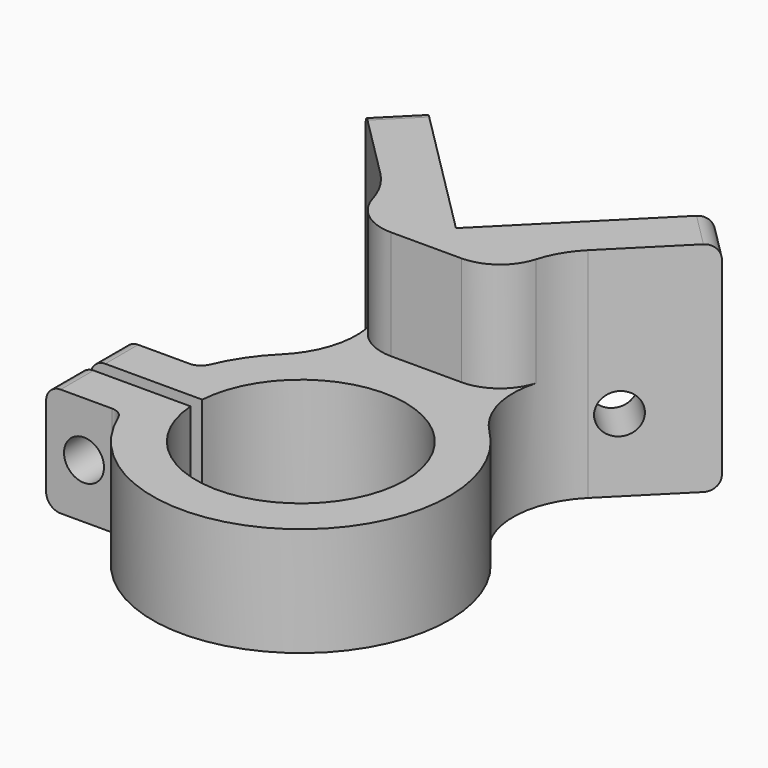
from build123d import *

# Parameters (mm, degrees)
F1_DEPTH      = 45
F2_R          = 4.125
F3_DEPTH      = 10
F4_R          = 4.125
F5_DEPTH      = 10
F6_R          = 4.125
F7_DEPTH      = 20
F9_DEPTH      = 3
F10_R         = 18
F11_W         = 72.4435358676
F11_H         = 36.0539390085
F12_DEPTH     = 100
F13_T1_DEPTH  = 22.5
F13_T6_DEPTH  = 22.5
F13_T12_DEPTH = 22.5
F13_T18_DEPTH = 22.5
F13_T25_DEPTH = 22.5
F13_T31_DEPTH = 22.5
F13_T34_DEPTH = 23.5
F13_T36_DEPTH = 23.5
F13_T38_DEPTH = 25
F13_T40_DEPTH = 25
F14_R         = 10


# Not quite as in the source:
# - a fillet or chamfer that OpenCascade refuses, or shapes differently, is made with other operations: its cross-section is extruded or revolved along the edge and cut away or added


with BuildPart() as f1:
    # F0 (on Top) → F1 (new body)
    with BuildSketch(Plane.XY):
        with BuildLine():
            Line((29.6984848098, 29.6984848098), (0, 0))
            Line((0, 0), (-29.6984848098, 29.6984848098))
            Line((-29.6984848098, 29.6984848098), (-36.7695526217, 22.627416998))
            Line((-36.7695526217, 22.627416998), (-4.4122546938, -9.7298809299))
            ThreePointArc((-4.4122546938, -9.7298809299), (-19.5013094439, -16.4320762481), (-28.9093081896, -30))
            ThreePointArc((-28.9093081896, -30), (-30.0334813831, -34.1915496034), (-30.5532011416, -38.5))
            Line((-30.5532011416, -38.5), (-21.53782951, -38.5))
            ThreePointArc((-21.53782951, -38.5), (21.59, -40), (-21.53782951, -41.5))
            Line((-21.53782951, -41.5), (-30.5532011416, -41.5))
            ThreePointArc((-30.5532011416, -41.5), (-30.0334813831, -45.8084503966), (-28.9093081896, -50))
            ThreePointArc((-28.9093081896, -50), (23.5679237519, -59.5013094439), (4.4122546938, -9.7298809299))
            Line((4.4122546938, -9.7298809299), (36.7695526217, 22.627416998))
            Line((36.7695526217, 22.627416998), (29.6984848098, 29.6984848098))
        make_face()
        with BuildLine():
            ThreePointArc((-30.5532011416, -38.5), (-30.0334813831, -34.1915496034), (-28.9093081896, -30))
            Line((-28.9093081896, -30), (-44.5532011416, -30))
            Line((-44.5532011416, -30), (-44.5532011416, -38.5))
            Line((-44.5532011416, -38.5), (-30.5532011416, -38.5))
        make_face()
        with BuildLine():
            Line((-44.5532011416, -50), (-28.9093081896, -50))
            ThreePointArc((-28.9093081896, -50), (-30.0334813831, -45.8084503966), (-30.5532011416, -41.5))
            Line((-30.5532011416, -41.5), (-44.5532011416, -41.5))
            Line((-44.5532011416, -41.5), (-44.5532011416, -50))
        make_face()
    extrude(amount=F1_DEPTH)

    # F2 (on face) → F3 (cut, through all)
    with BuildSketch(Plane(origin=(0, 0, 0), x_dir=(-0.7071067812, -0.7071067812, 0), z_dir=(-0.7071067812, 0.7071067812, 0))):
        with Locations((-25.4, 15)):
            Circle(F2_R)
    extrude(amount=-F3_DEPTH, mode=Mode.SUBTRACT)

    # F4 (on face) → F5 (cut, through all)
    with BuildSketch(Plane(origin=(0, 0, 0), x_dir=(-0.7071067812, 0.7071067812, 0), z_dir=(0.7071067812, 0.7071067812, 0))):
        with Locations((25.4, 15)):
            Circle(F4_R)
    extrude(amount=-F5_DEPTH, mode=Mode.SUBTRACT)

    # F6 (on face) → F7 (cut, through all)
    with BuildSketch(Plane.XZ.offset(50)):
        with Locations((-36.7312546656, 33.75)):
            Circle(F6_R)
        with Locations((-36.7312546656, 11.25)):
            Circle(F6_R)
    extrude(amount=-F7_DEPTH, mode=Mode.SUBTRACT)

    # F8 (on face) → F9 (cut)
    with BuildSketch(Plane(origin=(0, -30, 0), x_dir=(-1, 0, 0), z_dir=(0, 1, 0))):
        Polygon((43.6562546656, 37.7481506141), (36.7312546656, 41.7463012283), (29.8062546656, 37.7481506141), (29.8062546656, 29.7518493859), (36.7312546656, 25.7536987717), (43.6562546656, 29.7518493859), align=None)
        Polygon((43.6562546656, 7.2518493859), (43.6562546656, 15.2481506141), (36.7312546656, 19.2463012283), (29.8062546656, 15.2481506141), (29.8062546656, 7.2518493859), (36.7312546656, 3.2536987717), align=None)
    extrude(amount=-F9_DEPTH, mode=Mode.SUBTRACT)

    # F10
    f10_edges = [f1.edges().sort_by_distance(p)[0] for p in [
        (-4.412255, -9.729881, 22.5),
        (4.412255, -9.729881, 22.5),
    ]]
    fillet(f10_edges, radius=F10_R)

    # F11 (on Right) → F12 (cut, symmetric)
    with BuildSketch(Plane.YZ):
        with Locations((-43.9025410381, 40.5269695042)):
            Rectangle(F11_W, F11_H)
    extrude(amount=F12_DEPTH, both=True, mode=Mode.SUBTRACT)

    # F13: fillet of radius 3 on 10 edges, made by hand

    # F13_s2 → F13_t1 (join)
    with BuildSketch(Plane.XY):
        with BuildLine():
            ThreePointArc((-28.206162374, -51.8389401608), (-29.3115301597, -50.5016826145), (-30.9723764022, -50))
            Line((-30.9723764022, -50), (-28.9093081896, -50))
            ThreePointArc((-28.9093081896, -50), (-28.5725334833, -50.9251283904), (-28.206162374, -51.8389401608))
        make_face()
    extrude(amount=F13_T1_DEPTH)


with BuildPart() as f13_tool4:
    # F13_s5 → F13_t6 (new body)
    with BuildSketch(Plane.XY):
        with BuildLine():
            ThreePointArc((-28.206162374, -28.1610598392), (-29.3115301597, -29.4983173855), (-30.9723764022, -30))
            Line((-30.9723764022, -30), (-28.9093081896, -30))
            ThreePointArc((-28.9093081896, -30), (-28.5725334833, -29.0748716096), (-28.206162374, -28.1610598392))
        make_face()
    extrude(amount=F13_T6_DEPTH)

    split(bisect_by=Plane(origin=(-10.5917065627, 0, 18.3453739054), x_dir=(0, 1, 0), z_dir=(0.5, 0, -0.8660254038)), keep=Keep.TOP)

    split(bisect_by=Plane.YZ.offset(-29.8062546656), keep=Keep.TOP)


with BuildPart() as f1_1:
    add(f1.part)

    # F13_t3: union F13_tool4
    add(f13_tool4.part)


with BuildPart() as f13_tool10:
    # F13_s11 → F13_t12 (new body)
    with BuildSketch(Plane.XY):
        with BuildLine():
            ThreePointArc((-28.206162374, -28.1610598392), (-29.3115301597, -29.4983173855), (-30.9723764022, -30))
            Line((-30.9723764022, -30), (-28.9093081896, -30))
            ThreePointArc((-28.9093081896, -30), (-28.5725334833, -29.0748716096), (-28.206162374, -28.1610598392))
        make_face()
    extrude(amount=F13_T12_DEPTH)

    split(bisect_by=Plane(origin=(-10.5917065627, 0, 18.3453739054), x_dir=(0, 1, 0), z_dir=(0.5, 0, -0.8660254038)), keep=Keep.TOP)

    split(bisect_by=Plane.YZ.offset(-29.8062546656), keep=Keep.BOTTOM)


with BuildPart() as f1_2:
    add(f1_1.part)

    # F13_t9: union F13_tool10
    add(f13_tool10.part)


with BuildPart() as f13_tool16:
    # F13_s17 → F13_t18 (new body)
    with BuildSketch(Plane.XY):
        with BuildLine():
            ThreePointArc((-28.206162374, -28.1610598392), (-29.3115301597, -29.4983173855), (-30.9723764022, -30))
            Line((-30.9723764022, -30), (-28.9093081896, -30))
            ThreePointArc((-28.9093081896, -30), (-28.5725334833, -29.0748716096), (-28.206162374, -28.1610598392))
        make_face()
    extrude(amount=F13_T18_DEPTH)

    split(bisect_by=Plane(origin=(-10.5917065627, 0, 18.3453739054), x_dir=(0, 1, 0), z_dir=(-0.5, 0, 0.8660254038)), keep=Keep.TOP)

    split(bisect_by=Plane.YZ.offset(-29.8062546656), keep=Keep.TOP)

    split(bisect_by=Plane(origin=(-0.8489207701, 0, -1.4703739054), x_dir=(0, 1, 0), z_dir=(-0.5, 0, -0.8660254038)), keep=Keep.TOP)


with BuildPart() as f1_3:
    add(f1_2.part)

    # F13_t15: union F13_tool16
    add(f13_tool16.part)


with BuildPart() as f13_tool23:
    # F13_s24 → F13_t25 (new body)
    with BuildSketch(Plane.XY):
        with BuildLine():
            ThreePointArc((-28.206162374, -28.1610598392), (-29.3115301597, -29.4983173855), (-30.9723764022, -30))
            Line((-30.9723764022, -30), (-28.9093081896, -30))
            ThreePointArc((-28.9093081896, -30), (-28.5725334833, -29.0748716096), (-28.206162374, -28.1610598392))
        make_face()
    extrude(amount=F13_T25_DEPTH)

    split(bisect_by=Plane.YZ.offset(-29.8062546656), keep=Keep.TOP)

    split(bisect_by=Plane(origin=(-0.8489207701, 0, -1.4703739054), x_dir=(0, 1, 0), z_dir=(0.5, 0, 0.8660254038)), keep=Keep.TOP)


with BuildPart() as f1_4:
    add(f1_3.part)

    # F13_t22: union F13_tool23
    add(f13_tool23.part)


with BuildPart() as f13_tool29:
    # F13_s30 → F13_t31 (new body)
    with BuildSketch(Plane.XY):
        with BuildLine():
            ThreePointArc((-28.206162374, -28.1610598392), (-29.3115301597, -29.4983173855), (-30.9723764022, -30))
            Line((-30.9723764022, -30), (-28.9093081896, -30))
            ThreePointArc((-28.9093081896, -30), (-28.5725334833, -29.0748716096), (-28.206162374, -28.1610598392))
        make_face()
    extrude(amount=F13_T31_DEPTH)

    split(bisect_by=Plane.YZ.offset(-29.8062546656), keep=Keep.BOTTOM)

    split(bisect_by=Plane(origin=(-0.8489207701, 0, -1.4703739054), x_dir=(0, 1, 0), z_dir=(0.5, 0, 0.8660254038)), keep=Keep.TOP)


with BuildPart() as f1_5:
    add(f1_4.part)

    # F13_t28: union F13_tool29
    add(f13_tool29.part)

    # F13_s35 → F13_t34 (cut)
    with BuildSketch(Plane.XZ.offset(34)):
        with BuildLine():
            ThreePointArc((-44.5532011416, 3), (-43.6745214852, 0.8786796564), (-41.5532011416, 0))
            Line((-41.5532011416, 0), (-44.5532011416, 0))
            Line((-44.5532011416, 0), (-44.5532011416, 3))
        make_face()
        with BuildLine():
            ThreePointArc((-44.5532011416, 19.5), (-43.6745214852, 21.6213203436), (-41.5532011416, 22.5))
            Line((-41.5532011416, 22.5), (-44.5532011416, 22.5))
            Line((-44.5532011416, 22.5), (-44.5532011416, 19.5))
        make_face()
    extrude(amount=F13_T34_DEPTH, mode=Mode.SUBTRACT)

    # F13_s37 → F13_t36 (cut)
    with BuildSketch(Plane.XZ.offset(22.5)):
        with BuildLine():
            ThreePointArc((-44.5532011416, 3), (-43.6745214852, 0.8786796564), (-41.5532011416, 0))
            Line((-41.5532011416, 0), (-44.5532011416, 0))
            Line((-44.5532011416, 0), (-44.5532011416, 3))
        make_face()
        with BuildLine():
            ThreePointArc((-44.5532011416, 19.5), (-43.6745214852, 21.6213203436), (-41.5532011416, 22.5))
            Line((-41.5532011416, 22.5), (-44.5532011416, 22.5))
            Line((-44.5532011416, 22.5), (-44.5532011416, 19.5))
        make_face()
    extrude(amount=F13_T36_DEPTH, mode=Mode.SUBTRACT)

    # F13_s39 → F13_t38 (cut)
    with BuildSketch(Plane(origin=(5.3033008589, 5.3033008589, 0), x_dir=(0, 0, 1), z_dir=(-0.7071067812, -0.7071067812, 0))):
        with BuildLine():
            ThreePointArc((42, 42), (44.1213203436, 41.1213203436), (45, 39))
            Line((45, 39), (45, 42))
            Line((45, 42), (42, 42))
        make_face()
        with BuildLine():
            ThreePointArc((3, 42), (0.8786796564, 41.1213203436), (0, 39))
            Line((0, 39), (0, 42))
            Line((0, 42), (3, 42))
        make_face()
    extrude(amount=F13_T38_DEPTH, mode=Mode.SUBTRACT)

    # F13_s41 → F13_t40 (cut)
    with BuildSketch(Plane(origin=(12.3743686708, -12.3743686708, 0), x_dir=(0, 0, 1), z_dir=(-0.7071067812, 0.7071067812, 0))):
        with BuildLine():
            ThreePointArc((45, 39), (44.1213203436, 41.1213203436), (42, 42))
            Line((42, 42), (45, 42))
            Line((45, 42), (45, 39))
        make_face()
        with BuildLine():
            ThreePointArc((3, 42), (0.8786796564, 41.1213203436), (0, 39))
            Line((0, 39), (0, 42))
            Line((0, 42), (3, 42))
        make_face()
    extrude(amount=F13_T40_DEPTH, mode=Mode.SUBTRACT)

    # F14
    f14_edges = [f1_5.edges().sort_by_distance(p)[0] for p in [
        (-16.296581, -7.680773, 33.75),
        (16.296581, -7.680773, 33.75),
    ]]
    fillet(f14_edges, radius=F14_R)


solid = f1_5.part
